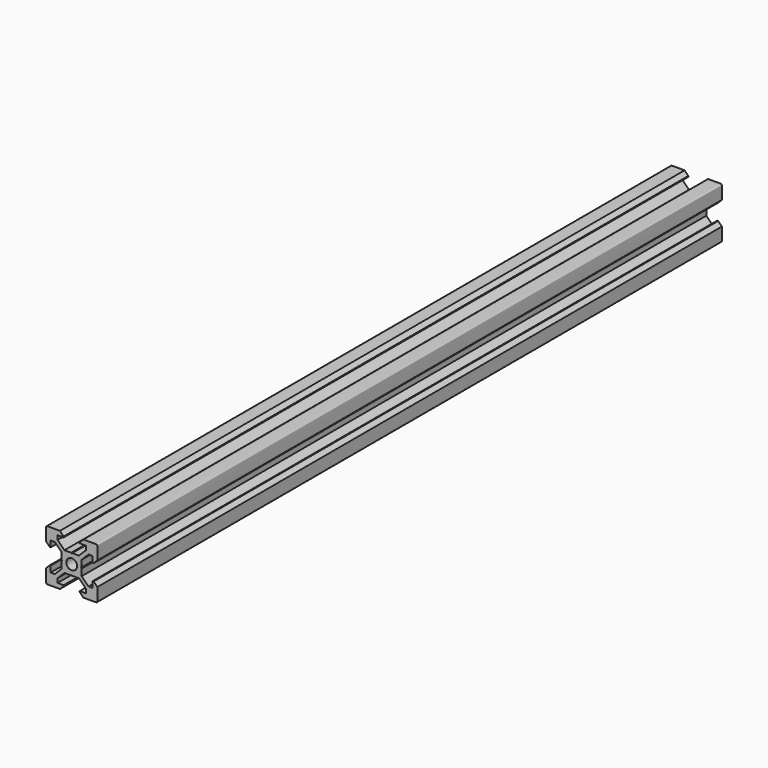
from build123d import *

# Parameters (mm, degrees)
F1_DEPTH = 304.8


# Not quite as in the source:
# - the dataset's text gives a spline's control points without its knots; the knots are read off the source's solid


with BuildPart() as f1:
    # F0 (on Front) → F1 (new body)
    with BuildSketch(Plane.XZ):
        with BuildLine():
            add(Edge.make_bspline(
                [(-8.545, 3.1250000004), (-8.43, 3.1250000004), (-8.315, 3.1250000004), (-8.2, 3.1250000004)],
                knots=[0, 0, 0, 0, 1, 1, 1, 1], degree=3))
            add(Edge.make_bspline(
                [(-8.2, 3.1250000004), (-8.2, 3.9166666671), (-8.2, 4.7083333338), (-8.2, 5.5000000004)],
                knots=[0, 0, 0, 0, 1, 1, 1, 1], degree=3))
            add(Edge.make_bspline(
                [(-8.1999999959, 5.5000000044), (-7.6535533893, 5.5000000044), (-7.1071067826, 5.5000000044), (-6.5606601759, 5.5000000044)],
                knots=[0, 0, 0, 0, 1, 1, 1, 1], degree=3))
            add(Edge.make_bspline(
                [(-6.5606601759, 5.5000000044), (-5.6737734493, 4.6131132778), (-4.7868867226, 3.7262265511), (-3.8999999959, 2.8393398244)],
                knots=[0, 0, 0, 0, 1, 1, 1, 1], degree=3))
            add(Edge.make_bspline(
                [(-3.8999999979, 2.8393398226), (-3.8999999979, 1.9628932159), (-3.8999999979, 1.0864466093), (-3.8999999979, 0.2100000026)],
                knots=[0, 0, 0, 0, 1, 1, 1, 1], degree=3))
            add(Edge.make_bspline(
                [(-3.9, 0.2100000008), (-3.83, 0.1400000008), (-3.76, 0.0700000008), (-3.69, 8e-10)],
                knots=[0, 0, 0, 0, 1, 1, 1, 1], degree=3))
            add(Edge.make_bspline(
                [(-3.9, -0.2099999992), (-3.83, -0.1399999992), (-3.76, -0.0699999992), (-3.69, 8e-10)],
                knots=[0, 0, 0, 0, 1, 1, 1, 1], degree=3))
            add(Edge.make_bspline(
                [(-3.8999999991, -2.839339821), (-3.8999999987, -1.9628932143), (-3.8999999984, -1.0864466077), (-3.899999998, -0.210000001)],
                knots=[0, 0, 0, 0, 1, 1, 1, 1], degree=3))
            add(Edge.make_bspline(
                [(-6.5606601782, -5.5000000017), (-5.6737734512, -4.6131132754), (-4.7868867241, -3.7262265491), (-3.8999999971, -2.8393398228)],
                knots=[0, 0, 0, 0, 1, 1, 1, 1], degree=3))
            add(Edge.make_bspline(
                [(-8.1999999982, -5.5000000011), (-7.6535533915, -5.5000000013), (-7.1071067849, -5.5000000015), (-6.5606601782, -5.5000000017)],
                knots=[0, 0, 0, 0, 1, 1, 1, 1], degree=3))
            add(Edge.make_bspline(
                [(-8.2000000012, -3.1249999971), (-8.2000000015, -3.9166666637), (-8.2000000019, -4.7083333304), (-8.2000000022, -5.4999999971)],
                knots=[0, 0, 0, 0, 1, 1, 1, 1], degree=3))
            add(Edge.make_bspline(
                [(-8.5450000012, -3.1249999969), (-8.4300000012, -3.124999997), (-8.3150000012, -3.124999997), (-8.2000000012, -3.1249999971)],
                knots=[0, 0, 0, 0, 1, 1, 1, 1], degree=3))
            add(Edge.make_bspline(
                [(-10.0000000018, -4.5799999963), (-9.5150000016, -4.0949999965), (-9.0300000014, -3.6099999967), (-8.5450000012, -3.1249999969)],
                knots=[0, 0, 0, 0, 1, 1, 1, 1], degree=3))
            add(Edge.make_bspline(
                [(-10.0000000038, -9.4999999963), (-10.0000000032, -7.8599999963), (-10.0000000025, -6.2199999963), (-10.0000000018, -4.5799999963)],
                knots=[0, 0, 0, 0, 1, 1, 1, 1], degree=3))
            add(Edge.make_bspline(
                [(-9.5000000039, -9.9999999965), (-9.5655199967, -9.9999999965), (-9.6293005688, -9.9873132519), (-9.6913417201, -9.9619397628), (-9.7513299005, -9.9374058943), (-9.8054004587, -9.9012771024), (-9.8535533945, -9.853553387), (-9.8995865416, -9.8079305653), (-9.9357153335, -9.7538600072), (-9.9619397702, -9.6913417126), (-9.9873132593, -9.6308520521), (-10.0000000039, -9.56707148), (-10.0000000038, -9.4999999963)],
                knots=[0, 0, 0, 0, 0.25, 0.25, 0.25, 0.5, 0.5, 0.5, 0.75, 0.75, 0.75, 1, 1, 1, 1], degree=3))
            add(Edge.make_bspline(
                [(-4.580000004, -9.9999999986), (-6.220000004, -9.9999999979), (-7.860000004, -9.9999999972), (-9.500000004, -9.9999999965)],
                knots=[0, 0, 0, 0, 1, 1, 1, 1], degree=3))
            Line((-4.580000004, -9.9999999986), (-3.1250000034, -8.5449999991))
            add(Edge.make_bspline(
                [(-3.1250000033, -8.1999999991), (-3.1250000033, -8.3149999991), (-3.1250000034, -8.4299999991), (-3.1250000034, -8.5449999991)],
                knots=[0, 0, 0, 0, 1, 1, 1, 1], degree=3))
            add(Edge.make_bspline(
                [(-5.5000000033, -8.1999999982), (-4.7083333366, -8.1999999985), (-3.91666667, -8.1999999988), (-3.1250000033, -8.1999999991)],
                knots=[0, 0, 0, 0, 1, 1, 1, 1], degree=3))
            add(Edge.make_bspline(
                [(-5.5000000066, -6.5606601742), (-5.5000000069, -7.1071067808), (-5.5000000071, -7.6535533875), (-5.5000000073, -8.1999999942)],
                knots=[0, 0, 0, 0, 1, 1, 1, 1], degree=3))
            add(Edge.make_bspline(
                [(-2.8393398255, -3.8999999953), (-3.7262265526, -4.7868867216), (-4.6131132796, -5.6737734479), (-5.5000000066, -6.5606601742)],
                knots=[0, 0, 0, 0, 1, 1, 1, 1], degree=3))
            add(Edge.make_bspline(
                [(-0.2100000015, -3.9000000003), (-1.0864466082, -3.9), (-1.9628932149, -3.8999999996), (-2.8393398215, -3.8999999993)],
                knots=[0, 0, 0, 0, 1, 1, 1, 1], degree=3))
            add(Edge.make_bspline(
                [(-1.5e-09, -3.6900000004), (-0.0700000015, -3.7600000004), (-0.1400000015, -3.8300000004), (-0.2100000015, -3.9000000003)],
                knots=[0, 0, 0, 0, 1, 1, 1, 1], degree=3))
            add(Edge.make_bspline(
                [(0.2099999985, -3.9000000005), (0.1399999985, -3.8300000005), (0.0699999985, -3.7600000005), (-1.5e-09, -3.6900000004)],
                knots=[0, 0, 0, 0, 1, 1, 1, 1], degree=3))
            add(Edge.make_bspline(
                [(2.8393398185, -3.9000000016), (1.9628932118, -3.9000000012), (1.0864466051, -3.9000000009), (0.2099999985, -3.9000000005)],
                knots=[0, 0, 0, 0, 1, 1, 1, 1], degree=3))
            add(Edge.make_bspline(
                [(5.4999999974, -6.5606601827), (4.6131132711, -5.6737734557), (3.7262265448, -4.7868867286), (2.8393398185, -3.9000000016)],
                knots=[0, 0, 0, 0, 1, 1, 1, 1], degree=3))
            add(Edge.make_bspline(
                [(5.4999999967, -8.2000000027), (5.4999999969, -7.653553396), (5.4999999971, -7.1071067894), (5.4999999974, -6.5606601827)],
                knots=[0, 0, 0, 0, 1, 1, 1, 1], degree=3))
            add(Edge.make_bspline(
                [(3.1249999967, -8.2000000017), (3.9166666634, -8.200000002), (4.70833333, -8.2000000024), (5.4999999967, -8.2000000027)],
                knots=[0, 0, 0, 0, 1, 1, 1, 1], degree=3))
            add(Edge.make_bspline(
                [(3.1249999966, -8.5450000017), (3.1249999966, -8.4300000017), (3.1249999967, -8.3150000017), (3.1249999967, -8.2000000017)],
                knots=[0, 0, 0, 0, 1, 1, 1, 1], degree=3))
            add(Edge.make_bspline(
                [(4.579999996, -10.0000000023), (4.0949999962, -9.5150000021), (3.6099999964, -9.0300000019), (3.1249999966, -8.5450000017)],
                knots=[0, 0, 0, 0, 1, 1, 1, 1], degree=3))
            add(Edge.make_bspline(
                [(9.499999996, -10.0000000043), (7.859999996, -10.0000000037), (6.219999996, -10.000000003), (4.579999996, -10.0000000023)],
                knots=[0, 0, 0, 0, 1, 1, 1, 1], degree=3))
            add(Edge.make_bspline(
                [(9.999999996, -9.5000000043), (9.999999996, -9.5655199971), (9.9873132515, -9.6293005692), (9.9619397623, -9.6913417205), (9.9374058938, -9.7513299009), (9.9012771019, -9.8054004591), (9.8535533866, -9.853553395), (9.8079305649, -9.899586542), (9.7538600068, -9.9357153339), (9.6913417122, -9.9619397706), (9.6308520517, -9.9873132598), (9.5670714797, -10.0000000043), (9.499999996, -10.0000000043)],
                knots=[0, 0, 0, 0, 0.25, 0.25, 0.25, 0.5, 0.5, 0.5, 0.75, 0.75, 0.75, 1, 1, 1, 1], degree=3))
            add(Edge.make_bspline(
                [(9.9999999981, -4.5800000043), (9.9999999974, -6.2200000043), (9.9999999967, -7.8600000043), (9.999999996, -9.5000000043)],
                knots=[0, 0, 0, 0, 1, 1, 1, 1], degree=3))
            add(Edge.make_bspline(
                [(8.5449999987, -3.1250000037), (9.0299999985, -3.6100000039), (9.5149999983, -4.0950000041), (9.9999999981, -4.5800000043)],
                knots=[0, 0, 0, 0, 1, 1, 1, 1], degree=3))
            add(Edge.make_bspline(
                [(8.1999999987, -3.1250000036), (8.3149999987, -3.1250000036), (8.4299999987, -3.1250000037), (8.5449999987, -3.1250000037)],
                knots=[0, 0, 0, 0, 1, 1, 1, 1], degree=3))
            add(Edge.make_bspline(
                [(8.1999999977, -5.5000000036), (8.199999998, -4.7083333369), (8.1999999983, -3.9166666703), (8.1999999987, -3.1250000036)],
                knots=[0, 0, 0, 0, 1, 1, 1, 1], degree=3))
            add(Edge.make_bspline(
                [(6.5606601777, -5.5000000019), (7.1071067843, -5.5000000022), (7.653553391, -5.5000000024), (8.1999999977, -5.5000000026)],
                knots=[0, 0, 0, 0, 1, 1, 1, 1], degree=3))
            add(Edge.make_bspline(
                [(3.8999999988, -2.8393398208), (4.7868867251, -3.7262265479), (5.6737734514, -4.6131132749), (6.5606601777, -5.5000000019)],
                knots=[0, 0, 0, 0, 1, 1, 1, 1], degree=3))
            add(Edge.make_bspline(
                [(3.8999999999, -0.2100000008), (3.8999999995, -1.0864466075), (3.8999999991, -1.9628932142), (3.8999999988, -2.8393398208)],
                knots=[0, 0, 0, 0, 1, 1, 1, 1], degree=3))
            add(Edge.make_bspline(
                [(3.69, -8e-10), (3.76, -0.0700000008), (3.8299999999, -0.1400000008), (3.8999999999, -0.2100000008)],
                knots=[0, 0, 0, 0, 1, 1, 1, 1], degree=3))
            add(Edge.make_bspline(
                [(3.69, -8e-10), (3.76, 0.0699999992), (3.83, 0.1399999992), (3.9, 0.2099999992)],
                knots=[0, 0, 0, 0, 1, 1, 1, 1], degree=3))
            add(Edge.make_bspline(
                [(3.9, 0.2099999992), (3.9, 1.0864466059), (3.9, 1.9628932126), (3.9, 2.8393398192)],
                knots=[0, 0, 0, 0, 1, 1, 1, 1], degree=3))
            add(Edge.make_bspline(
                [(3.9, 2.8393398192), (4.7868867266, 3.7262265459), (5.6737734533, 4.6131132726), (6.5606601799, 5.4999999992)],
                knots=[0, 0, 0, 0, 1, 1, 1, 1], degree=3))
            add(Edge.make_bspline(
                [(6.5606601799, 5.4999999992), (7.1071067866, 5.4999999992), (7.6535533933, 5.4999999992), (8.2, 5.4999999992)],
                knots=[0, 0, 0, 0, 1, 1, 1, 1], degree=3))
            add(Edge.make_bspline(
                [(8.2, 5.5000000002), (8.2, 4.7083333336), (8.2, 3.9166666669), (8.2, 3.1250000002)],
                knots=[0, 0, 0, 0, 1, 1, 1, 1], degree=3))
            add(Edge.make_bspline(
                [(8.2, 3.1250000002), (8.315, 3.1250000002), (8.43, 3.1250000002), (8.545, 3.1250000002)],
                knots=[0, 0, 0, 0, 1, 1, 1, 1], degree=3))
            add(Edge.make_bspline(
                [(8.545, 3.1250000002), (9.03, 3.6100000002), (9.515, 4.0950000002), (10, 4.5800000002)],
                knots=[0, 0, 0, 0, 1, 1, 1, 1], degree=3))
            add(Edge.make_bspline(
                [(10, 4.5800000002), (10, 6.2200000002), (10, 7.8600000002), (10, 9.5000000002)],
                knots=[0, 0, 0, 0, 1, 1, 1, 1], degree=3))
            add(Edge.make_bspline(
                [(10, 9.5000000002), (10, 9.565519993), (9.9873132554, 9.6293005651), (9.9619397663, 9.6913417164), (9.9374058978, 9.7513298969), (9.901277106, 9.805400455), (9.8535533907, 9.8535533909), (9.807930569, 9.899586538), (9.7538600108, 9.9357153299), (9.6913417163, 9.9619397666), (9.6308520558, 9.9873132558), (9.5670714838, 10.0000000004), (9.5, 10.0000000004)],
                knots=[0, 0, 0, 0, 0.25, 0.25, 0.25, 0.5, 0.5, 0.5, 0.75, 0.75, 0.75, 1, 1, 1, 1], degree=3))
            add(Edge.make_bspline(
                [(9.5, 10.0000000004), (7.86, 10.0000000004), (6.22, 10.0000000004), (4.58, 10.0000000004)],
                knots=[0, 0, 0, 0, 1, 1, 1, 1], degree=3))
            add(Edge.make_bspline(
                [(4.58, 10.0000000004), (4.095, 9.5150000004), (3.61, 9.0300000004), (3.125, 8.5450000004)],
                knots=[0, 0, 0, 0, 1, 1, 1, 1], degree=3))
            add(Edge.make_bspline(
                [(3.125, 8.5450000004), (3.125, 8.4300000004), (3.125, 8.3150000004), (3.125, 8.2000000004)],
                knots=[0, 0, 0, 0, 1, 1, 1, 1], degree=3))
            add(Edge.make_bspline(
                [(3.125, 8.2000000004), (3.9166666667, 8.2000000004), (4.7083333334, 8.2000000004), (5.5, 8.2000000004)],
                knots=[0, 0, 0, 0, 1, 1, 1, 1], degree=3))
            add(Edge.make_bspline(
                [(5.5, 8.2000000004), (5.5, 7.6535533938), (5.5, 7.1071067871), (5.5, 6.5606601804)],
                knots=[0, 0, 0, 0, 1, 1, 1, 1], degree=3))
            add(Edge.make_bspline(
                [(5.5, 6.5606601804), (4.6131132734, 5.6737734538), (3.7262265467, 4.7868867271), (2.8393398201, 3.9000000004)],
                knots=[0, 0, 0, 0, 1, 1, 1, 1], degree=3))
            add(Edge.make_bspline(
                [(2.8393398201, 3.9000000004), (1.9628932134, 3.9000000004), (1.0864466067, 3.9000000004), (0.21, 3.9000000004)],
                knots=[0, 0, 0, 0, 1, 1, 1, 1], degree=3))
            add(Edge.make_bspline(
                [(0.21, 3.9000000004), (0.14, 3.8300000004), (0.07, 3.7600000004), (0, 3.6900000004)],
                knots=[0, 0, 0, 0, 1, 1, 1, 1], degree=3))
            add(Edge.make_bspline(
                [(0, 3.6900000004), (-0.07, 3.7600000004), (-0.14, 3.8300000004), (-0.21, 3.9000000004)],
                knots=[0, 0, 0, 0, 1, 1, 1, 1], degree=3))
            add(Edge.make_bspline(
                [(-0.21, 3.9000000004), (-1.0864466066, 3.9000000004), (-1.9628932133, 3.9000000004), (-2.8393398199, 3.9000000004)],
                knots=[0, 0, 0, 0, 1, 1, 1, 1], degree=3))
            add(Edge.make_bspline(
                [(-2.8393398239, 3.8999999964), (-3.7262265506, 4.7868867231), (-4.6131132773, 5.6737734498), (-5.5000000039, 6.5606601764)],
                knots=[0, 0, 0, 0, 1, 1, 1, 1], degree=3))
            add(Edge.make_bspline(
                [(-5.5, 6.5606601804), (-5.5, 7.1071067871), (-5.5, 7.6535533938), (-5.5, 8.2000000004)],
                knots=[0, 0, 0, 0, 1, 1, 1, 1], degree=3))
            add(Edge.make_bspline(
                [(-5.5, 8.2000000004), (-4.7083333333, 8.2000000004), (-3.9166666666, 8.2000000004), (-3.125, 8.2000000004)],
                knots=[0, 0, 0, 0, 1, 1, 1, 1], degree=3))
            add(Edge.make_bspline(
                [(-3.125, 8.2000000004), (-3.125, 8.3150000004), (-3.125, 8.4300000004), (-3.125, 8.5450000004)],
                knots=[0, 0, 0, 0, 1, 1, 1, 1], degree=3))
            Line((-3.125, 8.5450000004), (-4.58, 10.0000000004))
            add(Edge.make_bspline(
                [(-4.58, 10.0000000004), (-6.22, 10.0000000004), (-7.86, 10.0000000004), (-9.5, 10.0000000004)],
                knots=[0, 0, 0, 0, 1, 1, 1, 1], degree=3))
            add(Edge.make_bspline(
                [(-9.4999999998, 10.0000000004), (-9.5655199926, 10.0000000005), (-9.6293005647, 9.9873132559), (-9.691341716, 9.9619397667), (-9.7513298965, 9.9374058983), (-9.8054004546, 9.9012771064), (-9.8535533905, 9.8535533911), (-9.8995865376, 9.8079305694), (-9.9357153295, 9.7538600112), (-9.9619397662, 9.6913417167), (-9.9873132554, 9.6308520562), (-10, 9.5670714842), (-10, 9.5000000004)],
                knots=[0, 0, 0, 0, 0.25, 0.25, 0.25, 0.5, 0.5, 0.5, 0.75, 0.75, 0.75, 1, 1, 1, 1], degree=3))
            add(Edge.make_bspline(
                [(-10, 9.5000000004), (-10, 7.8600000004), (-10, 6.2200000004), (-10, 4.5800000004)],
                knots=[0, 0, 0, 0, 1, 1, 1, 1], degree=3))
            add(Edge.make_bspline(
                [(-10, 4.5800000004), (-9.515, 4.0950000004), (-9.03, 3.6100000004), (-8.545, 3.1250000004)],
                knots=[0, 0, 0, 0, 1, 1, 1, 1], degree=3))
        make_face()
        with BuildLine():
            add(Edge.make_bspline(
                [(2.1, -4e-10), (2.1000000002, 0.2748893568), (1.9906569307, 0.8245399239), (1.5235828541, 1.5235874774), (0.8245570992, 1.9906556095), (5e-10, 2.1546721958), (-0.8245570982, 1.9906556098), (-1.5235828533, 1.523587478), (-1.9906569302, 0.8245399247), (-2.1, 0.2748893577), (-2.1, 4e-10)],
                knots=[-3.1415926536, -3.1415926536, -3.1415926536, -3.1415926536, -2.7488935719, -2.3561944902, -1.9634954085, -1.5707963268, -1.1780972451, -0.7853981634, -0.3926990817, 0, 0, 0, 0], degree=3))
            add(Edge.make_bspline(
                [(2.1, -4e-10), (2.1, -0.2748893577), (1.9906569304, -0.8245399247), (1.5235828534, -1.523587478), (0.8245570983, -1.9906556098), (-4e-10, -2.1546721958), (-0.824557099, -1.9906556095), (-1.5235828539, -1.5235874774), (-1.9906569306, -0.8245399239), (-2.1, -0.2748893568), (-2.1, 4e-10)],
                knots=[-3.1415926536, -3.1415926536, -3.1415926536, -3.1415926536, -2.7488935719, -2.3561944902, -1.9634954085, -1.5707963268, -1.1780972451, -0.7853981634, -0.3926990817, 0, 0, 0, 0], degree=3))
        make_face(mode=Mode.SUBTRACT)
    extrude(amount=-F1_DEPTH)


solid = f1.part
